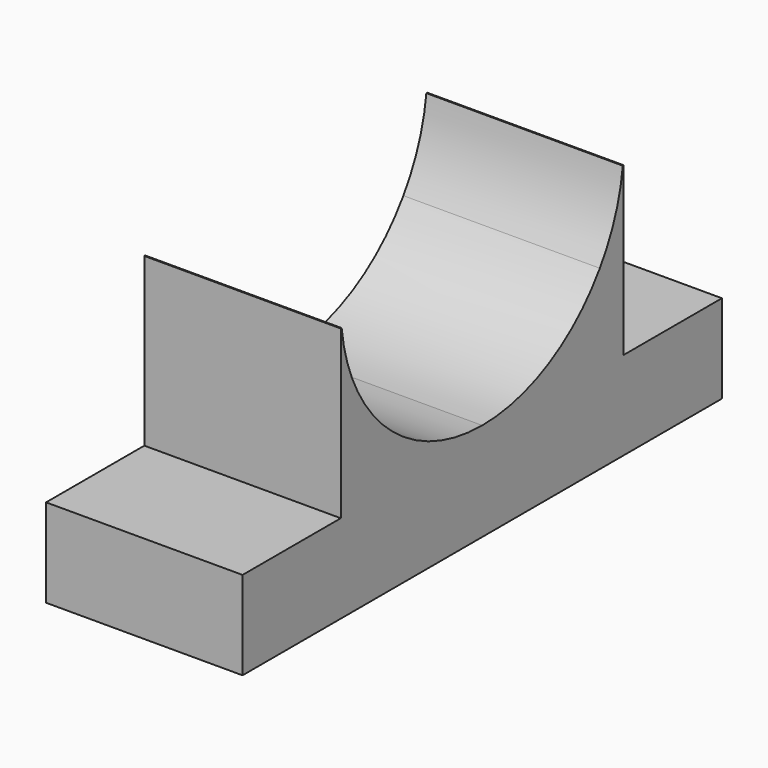
from build123d import *

# Parameters (mm, degrees)
F1_DEPTH = 20


with BuildPart() as f1:
    # F0 (on Right) → F1 (new body)
    with BuildSketch(Plane.YZ):
        with BuildLine():
            Line((18, -2), (17.88854382, -2))
            ThreePointArc((17.88854382, -2), (16.9075605646, -6.1753053167), (14.9666295471, -10))
            Line((14.9666295471, -10), (18, -10))
            Line((18, -10), (18, -2))
        make_face()
        with BuildLine():
            Line((18, -10), (14.9666295471, -10))
            ThreePointArc((14.9666295471, -10), (8.4852813742, -15.8745078664), (0, -18))
            Line((0, -18), (14.3178210633, -18))
            ThreePointArc((14.3178210633, -18), (16.2634559673, -16.2634559673), (18, -14.3178210633))
            Line((18, -14.3178210633), (18, -10))
        make_face()
        with BuildLine():
            Line((-14.3178210633, -18), (0, -18))
            ThreePointArc((0, -18), (-8.4852813742, -15.8745078664), (-14.9666295471, -10))
            Line((-14.9666295471, -10), (-18, -10))
            Line((-18, -10), (-18, -14.3178210633))
            ThreePointArc((-18, -14.3178210633), (-16.2634559673, -16.2634559673), (-14.3178210633, -18))
        make_face()
        with BuildLine():
            Line((14.3178210633, -18), (0, -18))
            Line((0, -18), (-14.3178210633, -18))
            ThreePointArc((-14.3178210633, -18), (0, -23), (14.3178210633, -18))
        make_face()
        with BuildLine():
            ThreePointArc((-14.9666295471, -10), (-16.9075605646, -6.1753053167), (-17.88854382, -2))
            Line((-17.88854382, -2), (-18, -2))
            Line((-18, -2), (-18, -10))
            Line((-18, -10), (-14.9666295471, -10))
        make_face()
        with BuildLine():
            Line((18, -18), (14.3178210633, -18))
            ThreePointArc((14.3178210633, -18), (0, -23), (-14.3178210633, -18))
            Line((-14.3178210633, -18), (-17, -18))
            Line((-17, -18), (-18, -18))
            Line((-18, -18), (-18, -19))
            Line((-18, -19), (-30.5, -19))
            Line((-30.5, -19), (-30.5, -28))
            Line((-30.5, -28), (30.5, -28))
            Line((30.5, -28), (30.5, -19))
            Line((30.5, -19), (18, -19))
            Line((18, -19), (18, -18))
        make_face()
        with BuildLine():
            ThreePointArc((18, -14.3178210633), (16.2634559673, -16.2634559673), (14.3178210633, -18))
            Line((14.3178210633, -18), (18, -18))
            Line((18, -18), (18, -14.3178210633))
        make_face()
        with BuildLine():
            Line((-17, -18), (-14.3178210633, -18))
            ThreePointArc((-14.3178210633, -18), (-16.2634559673, -16.2634559673), (-18, -14.3178210633))
            Line((-18, -14.3178210633), (-18, -18))
            Line((-18, -18), (-17, -18))
        make_face()
    extrude(amount=F1_DEPTH)


solid = f1.part
